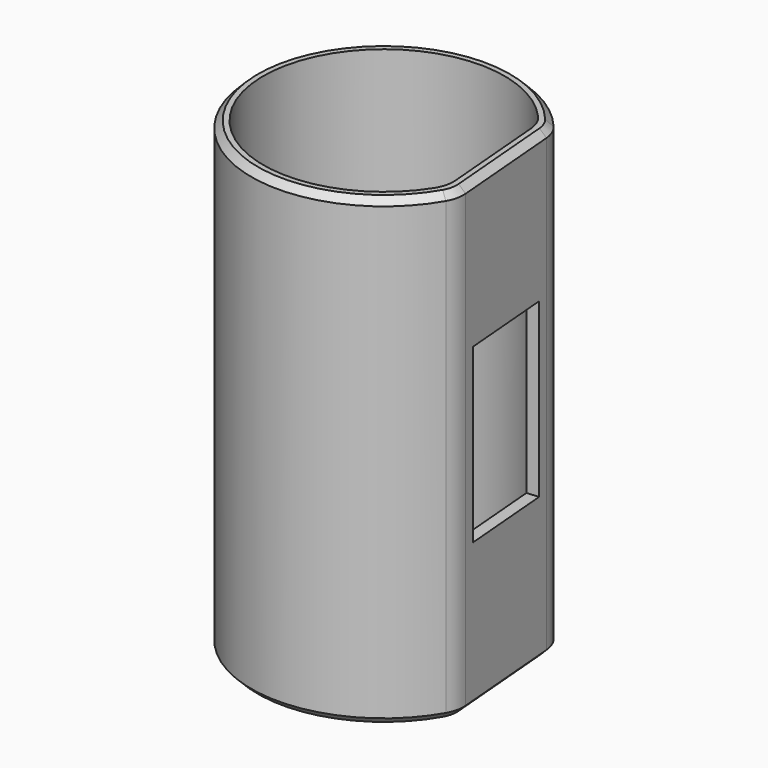
from build123d import *

# Parameters (mm, degrees)
F1_DEPTH = 70
F2_DEPTH = 2
F3_R     = 5
F4_SIZE  = 1
F5_W     = 14
F5_H     = 26
F6_DEPTH = 1.8


with BuildPart() as f1:
    # F0 (on Top) → F1 (new body)
    with BuildSketch(Plane.XY):
        with BuildLine():
            Line((18.100102838, -8.5080125325), (16.4182064079, 11.4211426026))
            ThreePointArc((16.4182064079, 11.4211426026), (-19.9291551351, -1.6818964302), (18.100102838, -8.5080125325))
        make_face()
        with BuildLine():
            ThreePointArc((16.264890885, -8.1665980983), (-18.1355311729, -1.5305257515), (14.6661704366, 10.776986811))
            Line((14.6661704366, 10.776986811), (16.264890885, -8.1665980983))
        make_face(mode=Mode.SUBTRACT)
    extrude(amount=F1_DEPTH)

    # F0 (on Top) → F2 (join)
    with BuildSketch(Plane.XY):
        with BuildLine():
            Line((16.264890885, -8.1665980983), (14.6661704366, 10.776986811))
            ThreePointArc((14.6661704366, 10.776986811), (-18.1355311729, -1.5305257515), (16.264890885, -8.1665980983))
        make_face()
    extrude(amount=F2_DEPTH)

    # F3
    f3_edges = [f1.edges().sort_by_distance(p)[0] for p in [
        (16.418206, 11.421143, 35),
        (14.66617, 10.776987, 36),
        (18.100103, -8.508013, 35),
        (16.264891, -8.166598, 36),
    ]]
    fillet(f3_edges, radius=F3_R)

    # F4
    f4_edges = [f1.edges().sort_by_distance(p)[0] for p in [
        (17.259155, 1.456565, 0),
        (17.876629, -8.57734, 0),
        (16.186274, 11.452037, 0),
        (-19.929155, -1.681896, 0),
        (-19.929155, -1.681896, 70),
        (17.259155, 1.456565, 70),
        (17.876629, -8.57734, 70),
        (16.186274, 11.452037, 70),
    ]]
    chamfer(f4_edges, length=F4_SIZE)

    # F5 (on face) → F6 (cut, through all)
    with BuildSketch(Plane(origin=(17.2591546229, 1.4565650351, 0), x_dir=(-0.0840948215, 0.9964577568, 0), z_dir=(0.9964577568, 0.0840948215, 0))):
        with Locations((0, 35)):
            Rectangle(F5_W, F5_H)
    extrude(amount=-F6_DEPTH, mode=Mode.SUBTRACT)


solid = f1.part
